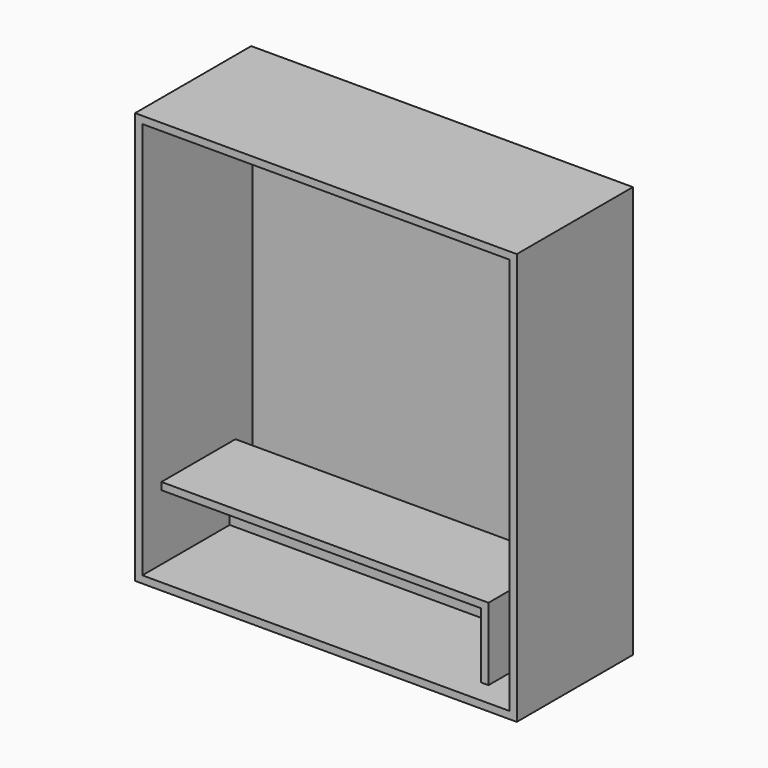
from build123d import *

# Parameters (mm, degrees)
F0_W          = 133.6063072085
F0_H          = 144.1496908665
F1_DEPTH      = 25.4
F1_DEPTH_BACK = 25.4
F2_T          = -2.54
F3_W          = 114.4931351459
F3_H          = 32.4011910707
F4_DEPTH      = 25.4
F5_T          = -2.54


# Not quite as in the source:
# - a shell that OpenCascade refuses in one call is made with other operations: the cavity is built on its own and cut out


with BuildPart() as f1:
    # F0 (on Front) → F1 (new body, two sides)
    with BuildSketch(Plane.XZ) as f1_sk:
        with Locations((-4.3567232788, -2.181828022)):
            Rectangle(F0_W, F0_H)
    extrude(amount=F1_DEPTH)
    extrude(f1_sk.sketch, amount=-F1_DEPTH_BACK)

    # F2
    f2_openings = [f1.faces().sort_by_distance(p)[0] for p in [
        (-4.356723, -25.4, -2.181828),
    ]]
    offset(amount=F2_T, openings=f2_openings)

    # F3 (on face) → F4 (join)
    with BuildSketch(Plane.XY.offset(-71.7166734552)):
        with Locations((-11.3733093101, -0.8654547855)):
            Rectangle(F3_W, F3_H)
    extrude(amount=F4_DEPTH)

    # F5: a shell. OpenCascade refuses it in one call, so the cavity is built on its own and cut out:
    # the body offset inwards by the wall thickness, plus a prism from it out through each open face.
    f5_core = offset(f1.part, amount=F5_T, kind=Kind.INTERSECTION, mode=Mode.PRIVATE)
    f5_exits = [f5_core.faces().sort_by_distance(p)[0] for p in [
        (-12.643309, -14.52605, -60.286673),
    ]]
    add(f5_core, mode=Mode.SUBTRACT)
    extrude(f5_exits, amount=-F5_T, mode=Mode.SUBTRACT)


solid = f1.part
